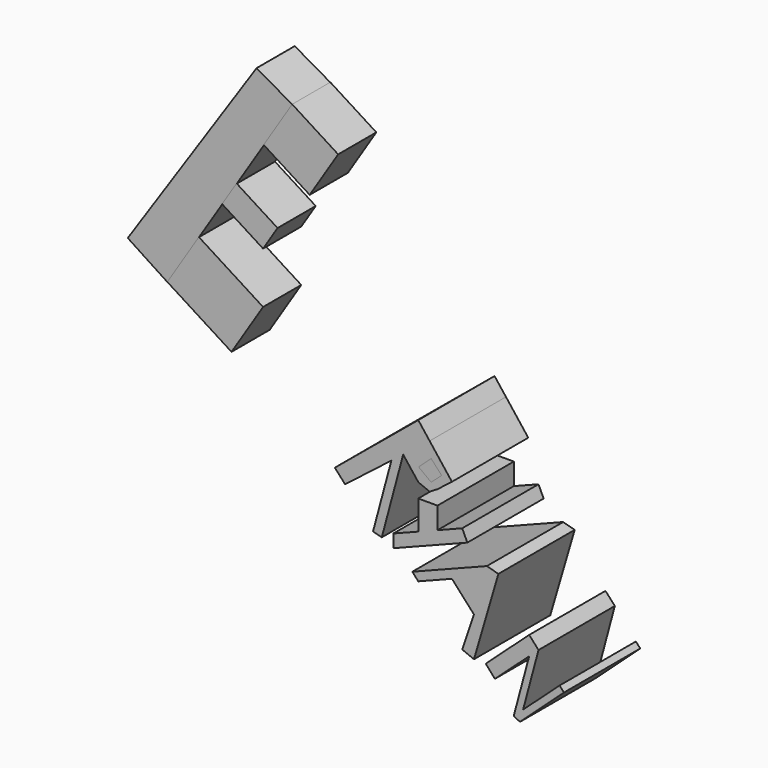
from build123d import *

# Parameters (mm, degrees)
F2_DEPTH = 25.4
F5_DEPTH = 50.8


with BuildPart() as f2:
    # F1 (on Front) → F2 (new body)
    with BuildSketch(Plane.XZ):
        Polygon((-200.7486671209, -72.8788375854), (-134.1392695904, 31.924854964), (-153.2281637192, 42.8873971105), (-221.8337059021, -59.0789616108), align=None)
    extrude(amount=F2_DEPTH)


with BuildPart() as f2b:
    # F0 (on Front) → F2, piece 2 (new body)
    with BuildSketch(Plane.XZ):
        Polygon((-134.2803835869, 32.1001149714), (-149.450007216, 8.1652749375), (-124.9612532579, -7.3554129034), (-109.7916296289, 16.5794271305), align=None)
    extrude(amount=F2_DEPTH)


with BuildPart() as f2c:
    # F0 (on Front) → F2, piece 3 (new body)
    with BuildSketch(Plane.XZ):
        Polygon((-142.0590088453, -28.450820074), (-163.8883034377, -14.6156666915), (-171.5970264872, -26.7785955529), (-149.7677318947, -40.6137489354), align=None)
    extrude(amount=F2_DEPTH)


with BuildPart() as f2d:
    # F0 (on Front) → F2, piece 4 (new body)
    with BuildSketch(Plane.XZ):
        Polygon((-149.7677318947, -67.9721375065), (-183.9674201976, -46.2967722627), (-200.7720470428, -72.8113427758), (-166.57235874, -94.4867080196), align=None)
    extrude(amount=F2_DEPTH)


with BuildPart() as f5:
    # F3 (on Front) → F5 (new body)
    with BuildSketch(Plane.XZ):
        Polygon((17.2187387786, -164.1581819836), (12.250800617, -158.6832260941), (-10.8956162127, -179.6861290932), (-6.0069423464, -185.2330088712), (12.250800617, -168.6660556679), align=None)
        Polygon((28.4437571682, -177.1399527788), (9.0159587106, -194.7686064703), (7.3233359407, -201.084989581), (30.7541404358, -179.6861290932), align=None)
        Polygon((9.0159587106, -194.7686064703), (17.2187387786, -164.1581819836), (12.250800617, -168.6660556679), (4.0480205491, -199.2764801546), align=None)
        Polygon((7.3233359407, -201.084989581), (9.0159587106, -194.7686064703), (4.0480205491, -199.2764801546), align=None)
    extrude(amount=F5_DEPTH)


with BuildPart() as f5b:
    # F3 (on Front) → F5, piece 2 (new body)
    with BuildSketch(Plane.XZ):
        Polygon((-28.8802379445, -100.2793381423), (-40.7517962158, -84.9945247173), (-54.8363216213, -95.9338315591), (-46.8156449497, -106.2605758387), (-40.7517962158, -108.7391674519), (-36.5811732513, -106.2605758387), align=None)
        Polygon((-66.2396103144, -138.487637043), (-54.8363216213, -95.9338315591), (-61.1383294086, -100.8285365577), (-70.8956203459, -137.2399501218), align=None)
        Polygon((-54.8363216213, -95.9338315591), (-40.7517962158, -84.9945247173), (-46.8156449497, -77.1872264321), (-91.2482365966, -113.9447018504), (-85.7818871737, -119.9689358473), (-61.1383294086, -100.8285365577), (-60.0946135819, -96.9336881972), align=None)
        Polygon((-61.1383294086, -100.8285365577), (-54.8363216213, -95.9338315591), (-60.0946135819, -96.9336881972), align=None)
    extrude(amount=F5_DEPTH)


with BuildPart() as f5c:
    # F3 (on Front) → F5, piece 3 (new body)
    with BuildSketch(Plane.XZ):
        Polygon((-46.8156449497, -129.4741981435), (-36.5811732513, -125.4654534497), (-36.5811732513, -113.9447018504), (-46.8156449497, -113.9447018504), (-46.8156449497, -120.3112053809), align=None)
        Polygon((-60.0946135819, -141.5711641312), (-20.6791479141, -126.1325031519), (-23.4221895759, -120.3112053809), (-36.5811732513, -125.4654534497), (-46.8156449497, -129.4741981435), (-60.0946135819, -134.6754431725), align=None)
    extrude(amount=F5_DEPTH)


with BuildPart() as f5d:
    # F3 (on Front) → F5, piece 4 (new body)
    with BuildSketch(Plane.XZ):
        Polygon((-28.8802379445, -145.7642225958), (-10.3028491139, -138.487637043), (-10.3028491139, -133.7581687008), (-49.9818195821, -149.3000419905), (-46.8156449497, -152.7893500067), align=None)
        Polygon((-17.157621035, -158.6832260941), (-10.3028491139, -138.487637043), (-28.8802379445, -145.7642225958), align=None)
        Polygon((-10.3028491139, -133.7581687008), (-10.3028491139, -138.487637043), (-17.157621035, -158.6832260941), (-23.4221895759, -177.1399527788), (-17.157621035, -179.6861290932), (-4.1395589314, -135.4097666355), align=None)
    extrude(amount=F5_DEPTH)


with BuildPart() as f5e:
    # F4 (on Front) → F5, piece 5 (new body)
    with BuildSketch(Plane.XZ):
        Polygon((-34.3966597908, -99.0771427751), (-39.9274900556, -92.9909944534), (-46.624712646, -99.0771427751), (-39.9274900556, -104.1033238342), align=None)
    extrude(amount=F5_DEPTH)


solid = Compound([f2.part, f2b.part, f2c.part, f2d.part, f5.part, f5b.part, f5c.part, f5d.part, f5e.part])
